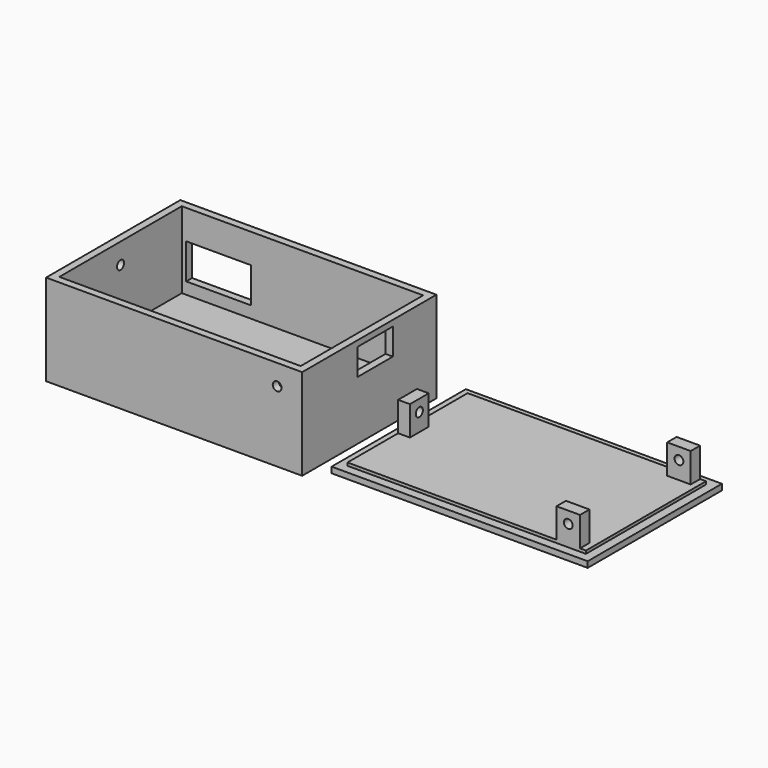
from build123d import *

# Parameters (mm, degrees)
F3_W      = 87
F3_H      = 57
F3_W_2    = 82
F3_H_2    = 52
F4_DEPTH  = 4
F3_R      = 1.5
F5_DEPTH  = 1
F7_R      = 4
F7_R_2    = 1.5
F8_DEPTH  = 3.5
F10_DEPTH = 27
F11_W     = 15
F11_H     = 9
F12_DEPTH = 2.5
F13_W     = 22
F13_H     = 12
F14_DEPTH = 2.5
F13_R     = 1.5
F15_DEPTH = 57.001
F3_W_3    = 81
F3_H_3    = 51
F18_DEPTH = 3
F19_DEPTH = 2
F20_W     = 8
F20_H     = 4
F20_W_2   = 4
F20_H_2   = 8
F21_DEPTH = 10
F22_R     = 1.5
F24_DEPTH = 54.001
F23_R     = 1.5
F25_DEPTH = 104.001
F26_R     = 1.5
F27_DEPTH = 2.5


with BuildPart() as f4:
    # F3 (on Top) → F4 (new body)
    with BuildSketch(Plane.XY):
        with Locations((43.5, 28.5)):
            Rectangle(F3_W, F3_H)
        with Locations((43.5, 28.5)):
            Rectangle(F3_W_2, F3_H_2, mode=Mode.SUBTRACT)
        with Locations((43.5, 28.5)):
            Rectangle(F3_W_2, F3_H_2)
        Polygon((6.625, 32.1950417228), (9.825, 30.3475208614), (9.825, 26.6524791386), (6.625, 24.8049582772), (3.425, 26.6524791386), (3.425, 30.3475208614), align=None, mode=Mode.SUBTRACT)
        Polygon((80.375, 32.1950417228), (83.575, 30.3475208614), (83.575, 26.6524791386), (80.375, 24.8049582772), (77.175, 26.6524791386), (77.175, 30.3475208614), align=None, mode=Mode.SUBTRACT)
    extrude(amount=-F4_DEPTH)

    # F3 (on Top) → F5 (join)
    with BuildSketch(Plane.XY):
        with Locations((43.5, 28.5)):
            Rectangle(F3_W, F3_H)
        with Locations((43.5, 28.5)):
            Rectangle(F3_W_2, F3_H_2, mode=Mode.SUBTRACT)
        with Locations((43.5, 28.5)):
            Rectangle(F3_W_2, F3_H_2)
        Polygon((6.625, 32.1950417228), (9.825, 30.3475208614), (9.825, 26.6524791386), (6.625, 24.8049582772), (3.425, 26.6524791386), (3.425, 30.3475208614), align=None, mode=Mode.SUBTRACT)
        Polygon((80.375, 32.1950417228), (83.575, 30.3475208614), (83.575, 26.6524791386), (80.375, 24.8049582772), (77.175, 26.6524791386), (77.175, 30.3475208614), align=None, mode=Mode.SUBTRACT)
        Polygon((9.825, 26.6524791386), (9.825, 30.3475208614), (6.625, 32.1950417228), (3.425, 30.3475208614), (3.425, 26.6524791386), (6.625, 24.8049582772), align=None)
        with Locations((6.625, 28.5)):
            Circle(F3_R, mode=Mode.SUBTRACT)
        Polygon((83.575, 26.6524791386), (83.575, 30.3475208614), (80.375, 32.1950417228), (77.175, 30.3475208614), (77.175, 26.6524791386), (80.375, 24.8049582772), align=None)
        with Locations((80.375, 28.5)):
            Circle(F3_R, mode=Mode.SUBTRACT)
    extrude(amount=F5_DEPTH)

    # F7 (on face) → F8 (join)
    with BuildSketch(Plane.XY.offset(1)):
        with Locations((6.625, 28.5)):
            Circle(F7_R)
        with Locations((6.625, 28.5)):
            Circle(F7_R_2, mode=Mode.SUBTRACT)
        with Locations((80.375, 28.5)):
            Circle(F7_R)
        with Locations((80.375, 28.5)):
            Circle(F7_R_2, mode=Mode.SUBTRACT)
    extrude(amount=F8_DEPTH)

    # F3 (on Top) → F10 (join)
    with BuildSketch(Plane.XY):
        with Locations((43.5, 28.5)):
            Rectangle(F3_W, F3_H)
        with Locations((43.5, 28.5)):
            Rectangle(F3_W_2, F3_H_2, mode=Mode.SUBTRACT)
    extrude(amount=F10_DEPTH)

    # F11 (on face) → F12 (cut, through all)
    with BuildSketch(Plane.YZ.offset(87)):
        with Locations((31, 20.5)):
            Rectangle(F11_W, F11_H)
    extrude(amount=-F12_DEPTH, mode=Mode.SUBTRACT)

    # F13 (on face) → F14 (cut)
    with BuildSketch(Plane(origin=(0, 57, 0), x_dir=(-1, 0, 0), z_dir=(0, 1, 0))):
        with Locations((-15, 11)):
            Rectangle(F13_W, F13_H)
    extrude(amount=-F14_DEPTH, mode=Mode.SUBTRACT)

    # F13 (on face) → F15 (cut, through all)
    with BuildSketch(Plane(origin=(0, 57, 0), x_dir=(-1, 0, 0), z_dir=(0, 1, 0))):
        with Locations((-78.5, 20)):
            Circle(F13_R)
    extrude(amount=-F15_DEPTH, mode=Mode.SUBTRACT)

    # F26 (on face) → F27 (cut, through all)
    with BuildSketch(Plane(origin=(0, 0, 0), x_dir=(0, -1, 0), z_dir=(-1, 0, 0))):
        with Locations((-28.5, 20)):
            Circle(F26_R)
    extrude(amount=-F27_DEPTH, mode=Mode.SUBTRACT)


with BuildPart() as f18:
    # F3 (on Top) → F18 (new body)
    with BuildSketch(Plane.XY):
        with Locations((140.5, 28.5)):
            Rectangle(F3_W_3, F3_H_3)
    extrude(amount=F18_DEPTH)

    # F3 (on Top) → F19 (join)
    with BuildSketch(Plane.XY):
        with Locations((140.5, 28.5)):
            Rectangle(F3_W, F3_H)
        with Locations((140.5, 28.5)):
            Rectangle(F3_W_3, F3_H_3, mode=Mode.SUBTRACT)
    extrude(amount=F19_DEPTH)

    # F20 (on face) → F21 (join)
    with BuildSketch(Plane.XY.offset(3)):
        with Locations((175, 52)):
            Rectangle(F20_W, F20_H)
        with Locations((175, 5)):
            Rectangle(F20_W, F20_H)
        with Locations((102, 28.5)):
            Rectangle(F20_W_2, F20_H_2)
    extrude(amount=F21_DEPTH)

    # F22 (on face) → F24 (cut, through all)
    with BuildSketch(Plane(origin=(0, 54, 0), x_dir=(-1, 0, 0), z_dir=(0, 1, 0))):
        with Locations((-175, 9)):
            Circle(F22_R)
    extrude(amount=-F24_DEPTH, mode=Mode.SUBTRACT)

    # F23 (on face) → F25 (cut, through all)
    with BuildSketch(Plane.YZ.offset(104)):
        with Locations((28.5, 9)):
            Circle(F23_R)
    extrude(amount=-F25_DEPTH, mode=Mode.SUBTRACT)


solid = Compound([f4.part, f18.part])
